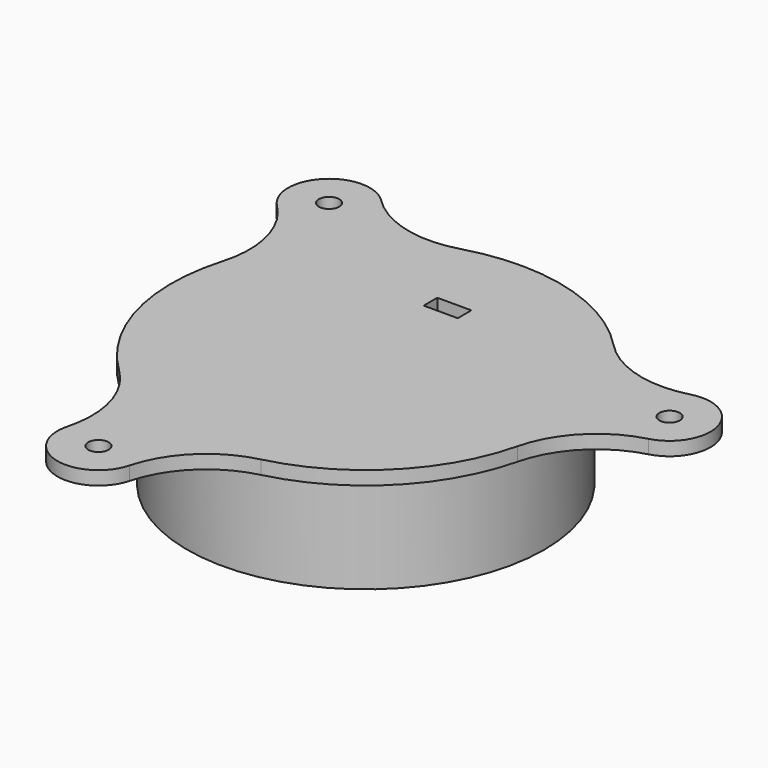
from build123d import *

# Parameters (mm, degrees)
F0_R     = 1.5
F1_DEPTH = 2
F3_DEPTH = 4
F2_W     = 5
F2_H     = 2.5
F4_DEPTH = 2.001
F7_R     = 4
F8_DEPTH = 5


# Not quite as in the source:
# - a feature names something its author has since deleted; it is built from what else it names


with BuildPart() as f1:
    # F0 (on Top) → F1 (new body)
    with BuildSketch(Plane.XY):
        with BuildLine():
            ThreePointArc((27.6844305044, -6.7692176539), (28.2953730261, -3.4090857003), (28.5, 0))
            ThreePointArc((28.5, 0), (26.4488952648, 10.6163053494), (20.5908112792, 19.7045297043))
            ThreePointArc((20.5908112792, 19.7045297043), (7.3763427854, 27.5288860492), (-7.9799008001, 27.3600289331))
            ThreePointArc((-7.9799008001, 27.3600289331), (-20.1525432638, 20.1525432638), (-27.3600289331, 7.9799008001))
            ThreePointArc((-27.3600289331, 7.9799008001), (-27.5288860492, -7.3763427854), (-19.7045297043, -20.5908112792))
            ThreePointArc((-19.7045297043, -20.5908112792), (-7.3763427854, -27.5288860492), (6.7692176539, -27.6844305044))
            ThreePointArc((6.7692176539, -27.6844305044), (20.1525432638, -20.1525432638), (27.6844305044, -6.7692176539))
        make_face()
        with BuildLine():
            ThreePointArc((20.5908112792, 19.7045297043), (26.4488952648, 10.6163053494), (28.5, 0))
            ThreePointArc((28.5, 0), (28.2953730261, -3.4090857003), (27.6844305044, -6.7692176539))
            ThreePointArc((27.6844305044, -6.7692176539), (31.4912676218, 0.0829769879), (38.2580956696, 4.0395687562))
            ThreePointArc((38.2580956696, 4.0395687562), (42.5007363567, 11.3880379845), (35.1522671284, 15.6306786716))
            ThreePointArc((35.1522671284, 15.6306786716), (27.3137262518, 15.6737736314), (20.5908112792, 19.7045297043))
        make_face()
        with Locations((36.705181399, 9.8351237139)):
            Circle(F0_R, mode=Mode.SUBTRACT)
        with BuildLine():
            ThreePointArc((-27.3600289331, 7.9799008001), (-20.1525432638, 20.1525432638), (-7.9799008001, 27.3600289331))
            ThreePointArc((-7.9799008001, 27.3600289331), (-15.8174939904, 27.2307492639), (-22.627416998, 31.1126983722))
            ThreePointArc((-22.627416998, 31.1126983722), (-31.1126983722, 31.1126983722), (-31.1126983722, 22.627416998))
            ThreePointArc((-31.1126983722, 22.627416998), (-27.2307492639, 15.8174939904), (-27.3600289331, 7.9799008001))
        make_face()
        with Locations((-26.8700576851, 26.8700576851)):
            Circle(F0_R, mode=Mode.SUBTRACT)
        with BuildLine():
            ThreePointArc((-4.0395687562, -38.2580956696), (-0.0829769879, -31.4912676218), (6.7692176539, -27.6844305044))
            ThreePointArc((6.7692176539, -27.6844305044), (-7.3763427854, -27.5288860492), (-19.7045297043, -20.5908112792))
            ThreePointArc((-19.7045297043, -20.5908112792), (-15.6737736314, -27.3137262518), (-15.6306786716, -35.1522671284))
            ThreePointArc((-15.6306786716, -35.1522671284), (-11.3880379845, -42.5007363567), (-4.0395687562, -38.2580956696))
        make_face()
        with Locations((-9.8351237139, -36.705181399)):
            Circle(F0_R, mode=Mode.SUBTRACT)
    extrude(amount=F1_DEPTH)

    # F2 (on Top) → F3 (join)
    with BuildSketch(Plane.XY):
        with BuildLine():
            Line((-4, -6.4), (-6.4, -6.4))
            Line((-6.4, -6.4), (-6.4, 6.4))
            Line((-6.4, 6.4), (-4, 6.4))
            Line((-4, 6.4), (-4, 10.246950766))
            ThreePointArc((-4, 10.246950766), (-11, 0), (-4, -10.246950766))
            Line((-4, -10.246950766), (-4, -6.4))
        make_face()
        with BuildLine():
            Line((4, 6.4), (6.4, 6.4))
            Line((6.4, 6.4), (6.4, -6.4))
            Line((6.4, -6.4), (4, -6.4))
            Line((4, -6.4), (4, -10.246950766))
            ThreePointArc((4, -10.246950766), (11, 0), (4, 10.246950766))
            Line((4, 10.246950766), (4, 6.4))
        make_face()
    extrude(amount=-F3_DEPTH)

    # F2 (on Top) → F4 (cut, through all)
    with BuildSketch(Plane.XY):
        with Locations((0, 15)):
            Rectangle(F2_W, F2_H)
    extrude(amount=F4_DEPTH, mode=Mode.SUBTRACT)


with BuildPart() as f6:
    # F5 (on Front) → F6 (revolve)
    with BuildSketch(Plane.XZ):
        with BuildLine():
            Line((22.6, 0), (14, 0))
            Line((14, 0), (13.4435483002, 0))
            ThreePointArc((13.4435483002, 0), (16.8052502032, -9.687101716), (26.2, -13.7955875195))
            Line((26.2, -13.7955875195), (26.2, -11.5))
            Line((26.2, -11.5), (26.2, -1))
            Line((26.2, -1), (25.2, -1))
            Line((25.2, -1), (25.2, -11.5))
            Line((25.2, -11.5), (22.6, -11.5))
            Line((22.6, -11.5), (22.6, 0))
        make_face()
        with BuildLine():
            ThreePointArc((25.2, -13.3551847397), (17.8707775672, -10.1801222006), (14, -3.1933057136))
            Line((14, -3.1933057136), (14, -1))
            Line((14, -1), (14.6787681728, -1))
            ThreePointArc((14.6787681728, -1), (17.7070613259, -8.7851638065), (25.2, -12.4777516446))
            Line((25.2, -12.4777516446), (25.2, -13.3551847397))
        make_face(mode=Mode.SUBTRACT)
        with BuildLine():
            ThreePointArc((21.8, -11.2138042548), (16.9098111592, -7.1134432734), (15.0787681728, -1))
            Line((15.0787681728, -1), (15.8787681728, -1))
            ThreePointArc((15.8787681728, -1), (17.4838871488, -6.5278570166), (21.8, -10.3363711597))
            Line((21.8, -10.3363711597), (21.8, -11.2138042548))
        make_face(mode=Mode.SUBTRACT)
        with BuildLine():
            Line((21.8, -9.0147455451), (21.8, -9.8921786402))
            ThreePointArc((21.8, -9.8921786402), (17.7713506121, -6.2334224428), (16.2787681728, -1))
            Line((16.2787681728, -1), (17.0569071889, -1))
            ThreePointArc((17.0569071889, -1), (18.3315263703, -5.6565297048), (21.8, -9.0147455451))
        make_face(mode=Mode.SUBTRACT)
        with BuildLine():
            ThreePointArc((21.8, -8.5552413531), (18.6200501231, -5.3572963828), (17.4569071889, -1))
            Line((17.4569071889, -1), (18.202930341, -1))
            ThreePointArc((18.202930341, -1), (19.1593952806, -4.7924936804), (21.8, -7.677808258))
            Line((21.8, -7.677808258), (21.8, -8.5552413531))
        make_face(mode=Mode.SUBTRACT)
        with BuildLine():
            Line((21.8, -6.3157460081), (21.8, -7.1931791032))
            ThreePointArc((21.8, -7.1931791032), (19.4493491461, -4.4848501334), (18.602930341, -1))
            Line((18.602930341, -1), (19.2994814961, -1))
            ThreePointArc((19.2994814961, -1), (19.9558252331, -3.9372499217), (21.8, -6.3157460081))
        make_face(mode=Mode.SUBTRACT)
        with BuildLine():
            ThreePointArc((21.8, -5.7850538993), (20.2477305909, -3.6128968026), (19.6994814961, -1))
            Line((19.6994814961, -1), (20.3153164614, -1))
            ThreePointArc((20.3153164614, -1), (20.6989951864, -3.0900828667), (21.8, -4.9076208042))
            Line((21.8, -4.9076208042), (21.8, -5.7850538993))
        make_face(mode=Mode.SUBTRACT)
        with BuildLine():
            Line((21.8, -1), (21.8, -4.2744088808))
            ThreePointArc((21.8, -4.2744088808), (20.9935443396, -2.7246950381), (20.7153164614, -1))
            Line((20.7153164614, -1), (21.8, -1))
        make_face(mode=Mode.SUBTRACT)
        with BuildLine():
            ThreePointArc((26.2, -13.7955875195), (16.8052502032, -9.687101716), (13.4435483002, 0))
            Line((13.4435483002, 0), (4, 0))
            Line((4, 0), (4, -7))
            Line((4, -7), (14, -7))
            ThreePointArc((14, -7), (19.0143728568, -12.5415234072), (26.2, -14.5955875195))
            Line((26.2, -14.5955875195), (26.2, -13.7955875195))
        make_face()
    revolve(axis=Axis((0, 0, -3.5), (0, 0, -1)))

    # F7 (on face) → F8 (cut)
    with BuildSketch(Plane(origin=(0, 0, 0), x_dir=(1, 0, 0), z_dir=(0, 0, -1))):
        with BuildLine():
            ThreePointArc((3.5, -10.8494239478), (0, 11.4), (-3.5, -10.8494239478))
            Line((-3.5, -10.8494239478), (-3.5, -16.6358047596))
            ThreePointArc((-3.5, -16.6358047596), (0, -17), (3.5, -16.6358047596))
            Line((3.5, -16.6358047596), (3.5, -10.8494239478))
        make_face()
        Circle(F7_R, mode=Mode.SUBTRACT)
    extrude(amount=F8_DEPTH, mode=Mode.SUBTRACT)


with BuildPart() as f10:
    # F9 (on Front) → F10 (revolve)
    with BuildSketch(Plane.XZ):
        with BuildLine():
            Line((14, -7.8), (3.3, -7.8))
            Line((3.3, -7.8), (3, -12))
            Line((3, -12), (0, -12))
            Line((0, -12), (0, -13))
            Line((0, -13), (1, -13))
            ThreePointArc((1, -13), (4.7710396279, -13.1994532812), (8.5, -13.7955875195))
            ThreePointArc((8.5, -13.7955875195), (12.9661214102, -12.372062791), (14, -7.8))
        make_face()
    revolve(axis=Axis((0, 0, -3.5), (0, 0, -1)))


solid = Compound([f1.part, f6.part, f10.part])
